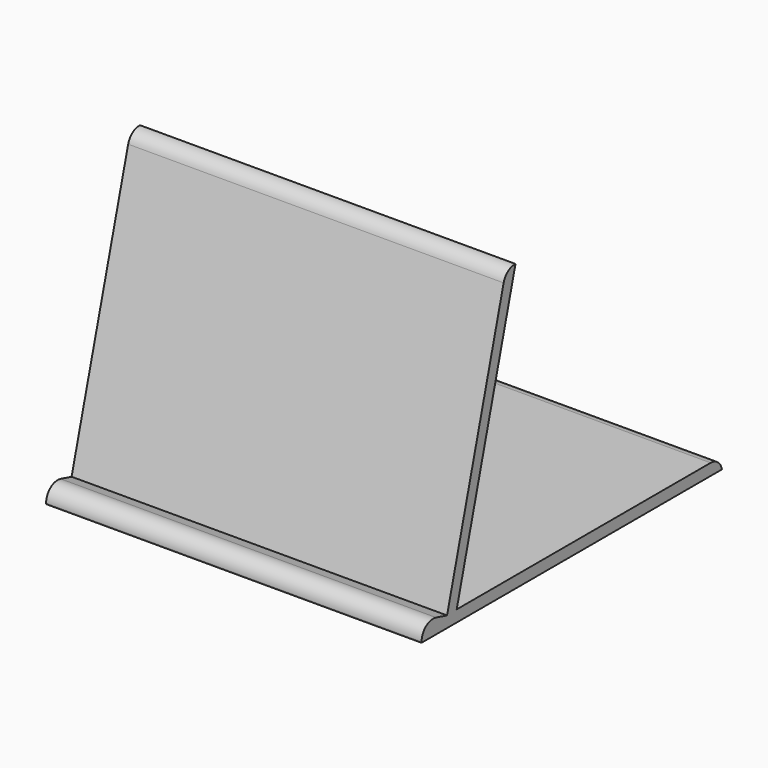
from build123d import *

# Parameters (mm, degrees)
F1_DEPTH    = 130
F2_T1_DEPTH = 154.4948974279
F3_T1_DEPTH = 154.4948974279
F4_R        = 5


# Not quite as in the source:
# - a fillet or chamfer that OpenCascade refuses, or shapes differently, is made with other operations: its cross-section is extruded or revolved along the edge and cut away or added


with BuildPart() as f1:
    # F0 (on Right) → F1 (new body)
    with BuildSketch(Plane.YZ):
        Polygon((1.0352761804, 3.8637033052), (0, 0), (120, 0), (120, 4), (5.2129014914, 4), (30.6586225483, 98.9647238196), (26.7949192431, 100), align=None)
        Polygon((-10, 0), (0, 0), (1.0352761804, 3.8637033052), (-10, 6.820596646), (-10, 4.0079755444), align=None)
    extrude(amount=F1_DEPTH)

    # F2: fillet of radius 5 on 1 edges, made by hand

    # F2_s2 → F2_t1 (cut)
    with BuildSketch(Plane.YZ.offset(-12.2474487139)):
        with BuildLine():
            ThreePointArc((30.6586225483, 98.9647238196), (27.4340422276, 98.0307814801), (25.5269700507, 95.2679491924))
            Line((25.5269700507, 95.2679491924), (26.7949192431, 100))
            Line((26.7949192431, 100), (30.6586225483, 98.9647238196))
        make_face()
    extrude(amount=F2_T1_DEPTH, mode=Mode.SUBTRACT)

    # F3: fillet of radius 5 on 1 edges, made by hand

    # F3_s2 → F3_t1 (cut)
    with BuildSketch(Plane.YZ.offset(-12.2474487139)):
        with BuildLine():
            ThreePointArc((115.1010205144, 4), (118.2632981746, 2.8729833462), (120, 0))
            Line((120, 0), (120, 4))
            Line((120, 4), (115.1010205144, 4))
        make_face()
    extrude(amount=F3_T1_DEPTH, mode=Mode.SUBTRACT)

    # F4
    f4_edges = [f1.edges().sort_by_distance(p)[0] for p in [
        (65, -10, 6.820597),
    ]]
    fillet(f4_edges, radius=F4_R)


solid = f1.part
